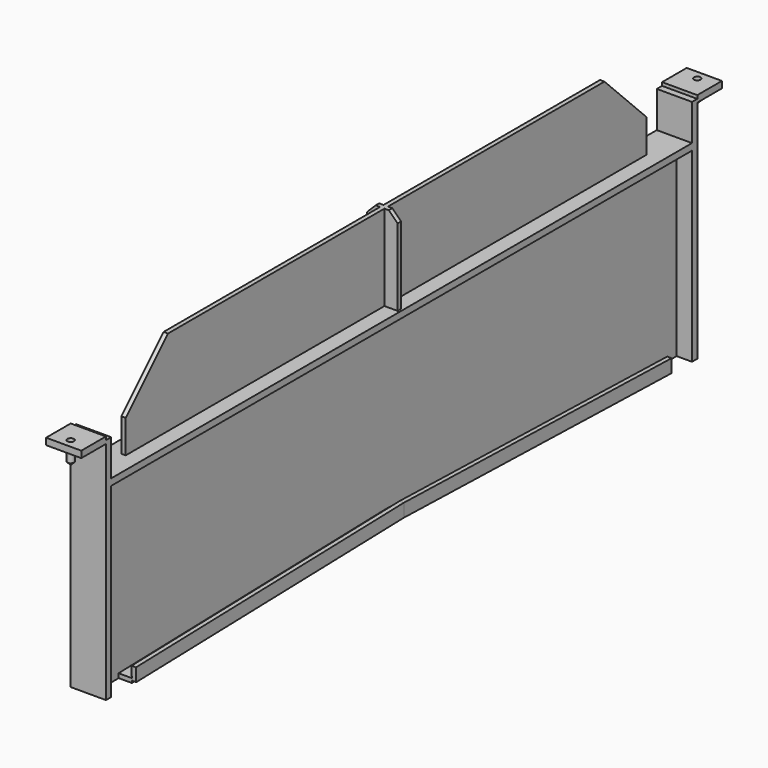
from build123d import *

# Parameters (mm, degrees)
F0_W      = 1047.75
F0_H      = 19.05
F1_DEPTH  = 50.8
F2_W      = 2095.5
F2_H      = 536.702
F3_DEPTH  = 6.35
F4_W      = 12.7
F4_H      = 1879.6
F5_DEPTH  = 247.65
F6_SIZE   = 152.4
F7_W      = 88.9
F7_H      = 12.7
F8_DEPTH  = 247.65
F9_SIZE   = 25.4
F11_D     = 19.05
F13_R     = 9.525
F14_DEPTH = 50.8
F15_SIZE  = 6.35
F18_DEPTH = 38.1
F20_DEPTH = 12.7


with BuildPart() as f1:
    # F0 (on Right) → F1 (new body, symmetric)
    with BuildSketch(Plane.YZ):
        Polygon((-1047.75, -9.525), (-1066.8, -9.525), (-1066.8, -19.05), (-1066.8, -669.925), (-1047.75, -669.925), (-1047.75, -133.223), (-1047.75, -114.173), align=None)
        Polygon((-1066.8, 0), (-1155.7, 0), (-1155.7, -19.05), (-1066.8, -19.05), (-1066.8, -9.525), align=None)
        with Locations((-523.875, -123.698)):
            Rectangle(F0_W, F0_H)
        with Locations((523.875, -123.698)):
            Rectangle(F0_W, F0_H)
        Polygon((1047.75, -9.525), (1047.75, -114.173), (1047.75, -133.223), (1047.75, -669.925), (1066.8, -669.925), (1066.8, -19.05), (1066.8, -9.525), align=None)
        Polygon((1066.8, 0), (1066.8, -9.525), (1066.8, -19.05), (1155.7, -19.05), (1155.7, 0), align=None)
    extrude(amount=F1_DEPTH, both=True)

    # F2 (on Right) → F3 (join, symmetric)
    with BuildSketch(Plane.YZ):
        with Locations((0, -401.574)):
            Rectangle(F2_W, F2_H)
    extrude(amount=F3_DEPTH, both=True)

    # F4 (on face) → F5 (join)
    with BuildSketch(Plane.XY.offset(-114.173)):
        Rectangle(F4_W, F4_H)
    extrude(amount=F5_DEPTH)

    # F6
    f6_edges = [f1.edges().sort_by_distance(p)[0] for p in [
        (0, -939.8, 133.477),
        (0, 939.8, 133.477),
    ]]
    chamfer(f6_edges, length=F6_SIZE)

    # F7 (on face) → F8 (join)
    with BuildSketch(Plane.XY.offset(-114.173)):
        Rectangle(F7_W, F7_H)
    extrude(amount=F8_DEPTH)

    # F9
    f9_edges = [f1.edges().sort_by_distance(p)[0] for p in [
        (44.45, 0, 133.477),
        (-44.45, 0, 133.477),
    ]]
    chamfer(f9_edges, length=F9_SIZE)

    # F11 (through all)
    with Locations(Plane.XY):
        with Locations((0, -1130.3), (0, 1130.3)):
            Hole(F11_D / 2)

    # F13 (on offset) → F14 (join)
    with BuildSketch(Plane.XY.offset(-9.525)):
        with Locations((0, -1130.3)):
            Circle(F13_R)
    extrude(amount=-F14_DEPTH)

    # F15
    f15_edges = [f1.edges().sort_by_distance(p)[0] for p in [
        (-9.525, -1130.3, -60.325),
    ]]
    chamfer(f15_edges, length=F15_SIZE)

    # F16: F1 across plane


with BuildPart() as f1_1:
    add(f1.part)
    add(f1.part.mirror(Plane.XZ))


with BuildPart() as f18:
    # F17 (on face) → F18 (new body)
    with BuildSketch(Plane.YZ.offset(6.35)):
        Polygon((-965.5340948625, -657.2293952242), (-965.2, -669.925), (0, -644.525), (-0.3340948625, -631.8293952242), align=None)
    extrude(amount=F18_DEPTH)

    # F19 (on face) → F20 (join)
    with BuildSketch(Plane.YZ.offset(44.45)):
        Polygon((-966.3693320188, -625.4903832848), (-965.3670474312, -663.5771976121), (0, -638.1728016271), (0, -600.0596113895), align=None)
    extrude(amount=F20_DEPTH)


with BuildPart() as f21_1:
    # F21: instance of F18
    add(f18.part.mirror(Plane.XZ))


with BuildPart() as f22_1:
    # F22: instance of F18
    add(f18.part.mirror(Plane.YZ))


with BuildPart() as f23_1:
    # F23: instance of F22_1
    add(f22_1.part.mirror(Plane.XZ))


solid = Compound([f1_1.part, f18.part, f21_1.part, f22_1.part, f23_1.part])
